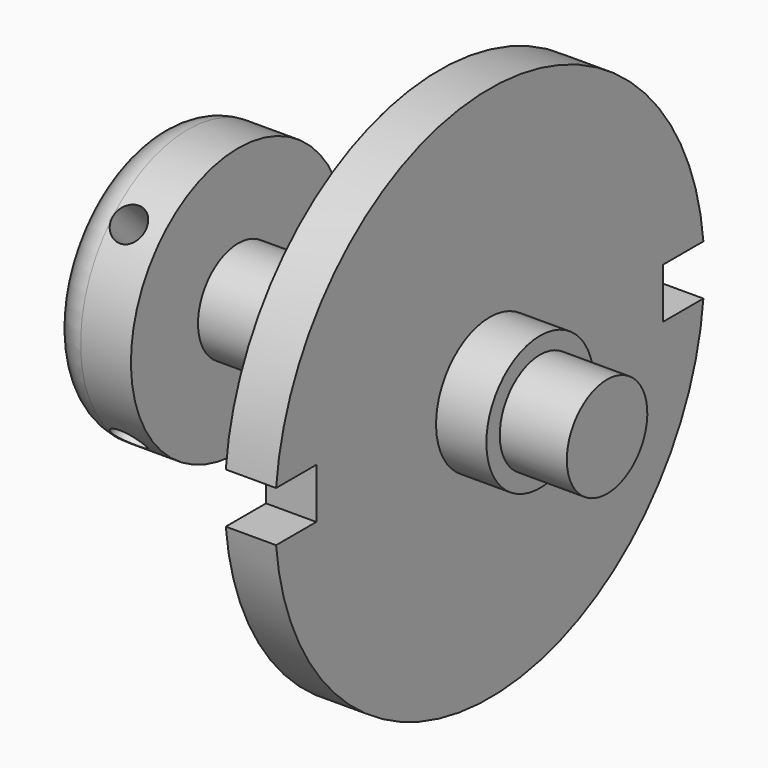
from build123d import *

# Parameters (mm, degrees)
F2_R             = 9.525
F3_DEPTH         = 20.828
F4_SIZE          = 5.08
F5_R             = 9.525
F6_DEPTH         = 20.828
F7_SIZE          = 5.08
F9_DEPTH         = 25.4
F11_DEPTH        = 25.4
F14_R            = 6.35
F15_DEPTH        = 25.4
F15_COPIES_COUNT = 4


# Not quite as in the source:
# - a pattern or mirror of a feature is missing from the dataset's text; its kind, count and spacing are read off the source's solid


with BuildPart() as f1:
    # F0 (on Front) → F1 (revolve)
    with BuildSketch(Plane.XZ):
        with BuildLine():
            Line((-171.45, 0), (0, 0))
            Line((0, 0), (0, 19.05))
            Line((0, 19.05), (-25.4, 19.05))
            Line((-25.4, 19.05), (-25.4, 25.4))
            Line((-25.4, 25.4), (-44.45, 25.4))
            Line((-44.45, 25.4), (-44.45, 101.6))
            Line((-44.45, 101.6), (-63.5, 101.6))
            Line((-63.5, 101.6), (-63.5, 19.05))
            Line((-63.5, 19.05), (-139.7, 19.05))
            Line((-139.7, 19.05), (-139.7, 50.8))
            Line((-139.7, 50.8), (-158.75, 50.8))
            ThreePointArc((-158.75, 50.8), (-167.7302561211, 47.0802561211), (-171.45, 38.1))
            Line((-171.45, 38.1), (-171.45, 0))
        make_face()
    revolve(axis=Axis((-33.1432974098, 0, 0), (1, 0, 0)))

    # F2 (on face) → F3 (join)
    with BuildSketch(Plane(origin=(-63.5, 0, 0), x_dir=(0, -1, 0), z_dir=(-1, 0, 0))):
        with Locations((0, 76.2)):
            Circle(F2_R)
    extrude(amount=F3_DEPTH)

    # F4
    f4_edges = [f1.edges().sort_by_distance(p)[0] for p in [
        (-84.328, 9.525, 76.2),
    ]]
    chamfer(f4_edges, length=F4_SIZE)

    # F5 (on face) → F6 (join)
    with BuildSketch(Plane(origin=(-63.5, 0, 0), x_dir=(0, -1, 0), z_dir=(-1, 0, 0))):
        with Locations((0, -76.2)):
            Circle(F5_R)
    extrude(amount=F6_DEPTH)

    # F7
    f7_edges = [f1.edges().sort_by_distance(p)[0] for p in [
        (-84.328, 9.525, -76.2),
    ]]
    chamfer(f7_edges, length=F7_SIZE)

    # F8 (on face) → F9 (cut)
    with BuildSketch(Plane(origin=(-63.5, 0, 0), x_dir=(0, -1, 0), z_dir=(-1, 0, 0))):
        with BuildLine():
            Line((-82.1025302452, 9.525), (-101.1525302452, 9.525))
            ThreePointArc((-101.1525302452, 9.525), (-101.6, 0), (-101.1525302452, -9.525))
            Line((-101.1525302452, -9.525), (-82.1025302452, -9.525))
            Line((-82.1025302452, -9.525), (-82.1025302452, 9.525))
        make_face()
    extrude(amount=-F9_DEPTH, mode=Mode.SUBTRACT)

    # F10 (on face) → F11 (cut)
    with BuildSketch(Plane(origin=(-63.5, 0, 0), x_dir=(0, -1, 0), z_dir=(-1, 0, 0))):
        with BuildLine():
            ThreePointArc((101.1525302452, -9.525), (101.6, 0), (101.1525302452, 9.525))
            Line((101.1525302452, 9.525), (82.1025302452, 9.525))
            Line((82.1025302452, 9.525), (82.1025302452, -9.525))
            Line((82.1025302452, -9.525), (101.1525302452, -9.525))
        make_face()
    extrude(amount=-F11_DEPTH, mode=Mode.SUBTRACT)

    # F14 (on line) → F15 (cut)
    with BuildSketch(Plane(origin=(0, -35.9210244843, 35.9210244843), x_dir=(1, 0, 0), z_dir=(0, -0.7071067812, 0.7071067812))):
        with Locations((-152.4, 0)):
            Circle(F14_R)
    f15 = extrude(amount=-F15_DEPTH, mode=Mode.SUBTRACT)

    # F15_copies: F15 ×4 about axis
    f15_copies_axis = Axis((0, 0, 0), (1, 0, 0))
    for i in range(1, F15_COPIES_COUNT):
        add(f15.rotate(f15_copies_axis, i * 360 / F15_COPIES_COUNT), mode=Mode.SUBTRACT)


solid = f1.part
